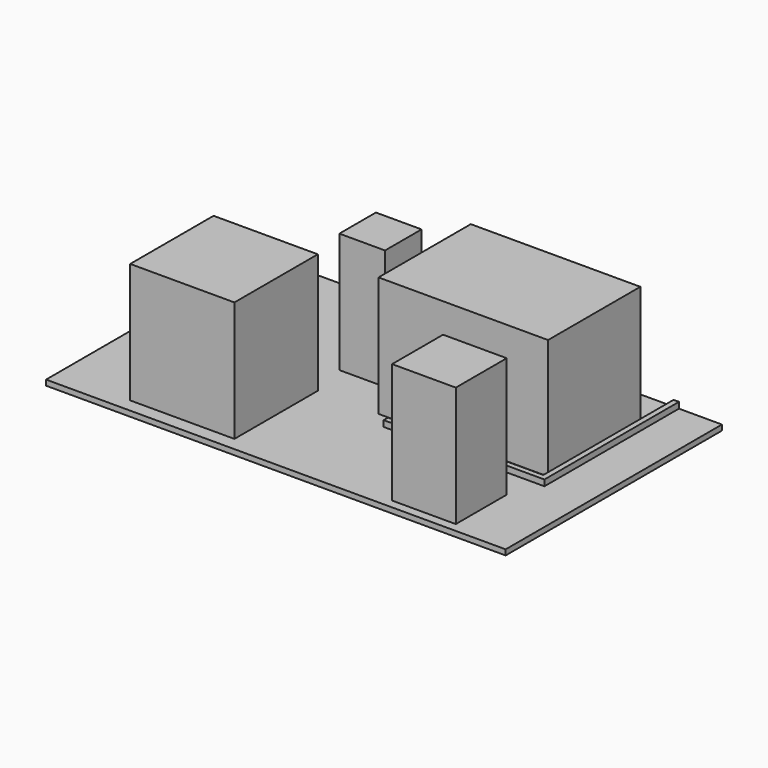
from build123d import *

# Parameters (mm, degrees)
F0_W     = 3470
F0_H     = 3470
F0_W_2   = 2120
F0_H_2   = 2120
F0_W_3   = 1520
F0_H_3   = 1520
F0_W_4   = 5645
F0_H_4   = 3840
F1_DEPTH = 180
F2_DEPTH = 4000
F3_DEPTH = 200


# Not quite as in the source:
# - a feature names something its author has since deleted; it is built from what else it names


with BuildPart() as f1:
    # F0 (on Top) → F1 (new body)
    with BuildSketch(Plane.XY):
        Polygon((-7650, 4500), (-7650, -4500), (7650, -4500), (7650, 4500), (6220, 4500), (6220, -1100), (870, -1100), (870, -920), (1050, -920), (6040, -920), (6040, 4500), align=None)
        with Locations((-3475, -2315)):
            Rectangle(F0_W, F0_H, mode=Mode.SUBTRACT)
        with Locations((4690, -3140)):
            Rectangle(F0_W_2, F0_H_2, mode=Mode.SUBTRACT)
        with Locations((-1270, 1440)):
            Rectangle(F0_W_3, F0_H_3, mode=Mode.SUBTRACT)
        with Locations((3127.5, 1310)):
            Rectangle(F0_W_4, F0_H_4, mode=Mode.SUBTRACT)
        Polygon((6220, 4500), (6040, 4500), (6040, -920), (1050, -920), (870, -920), (870, -1100), (6220, -1100), align=None)
        with Locations((-3475, -2315)):
            Rectangle(F0_W, F0_H)
        with Locations((-1270, 1440)):
            Rectangle(F0_W_3, F0_H_3)
        with Locations((4690, -3140)):
            Rectangle(F0_W_2, F0_H_2)
        with Locations((3127.5, 1310)):
            Rectangle(F0_W_4, F0_H_4)
    extrude(amount=-F1_DEPTH)

    # F0 (on Top) → F2 (join)
    with BuildSketch(Plane.XY):
        with Locations((-3475, -2315)):
            Rectangle(F0_W, F0_H)
        with Locations((-1270, 1440)):
            Rectangle(F0_W_3, F0_H_3)
        with Locations((4690, -3140)):
            Rectangle(F0_W_2, F0_H_2)
        with Locations((3127.5, 1310)):
            Rectangle(F0_W_4, F0_H_4)
    extrude(amount=F2_DEPTH)

    # F0 (on Top) → F3 (join)
    with BuildSketch(Plane.XY):
        Polygon((6220, 4500), (6040, 4500), (6040, -920), (1050, -920), (870, -920), (870, -1100), (6220, -1100), align=None)
    extrude(amount=F3_DEPTH)


solid = f1.part
